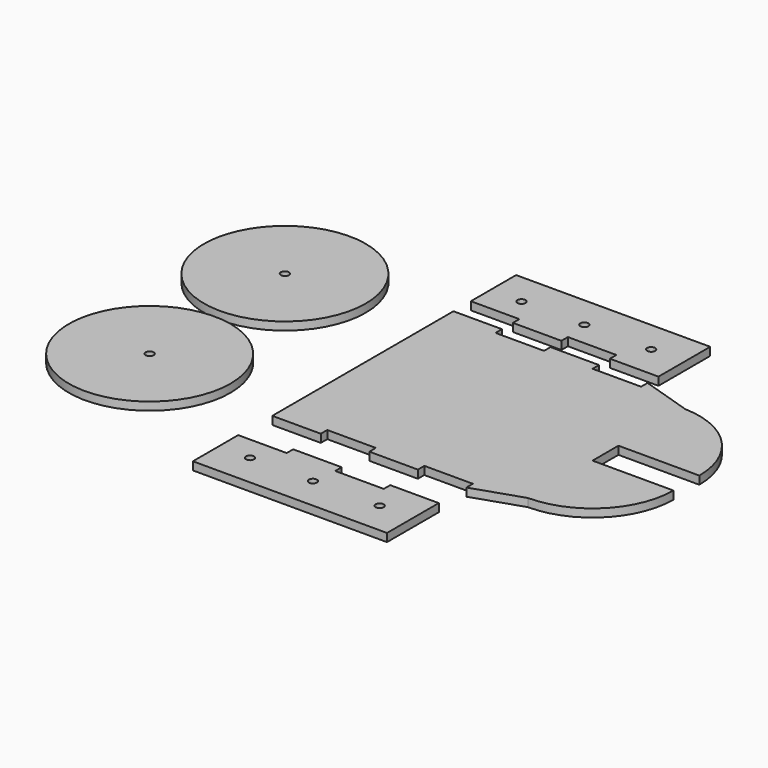
from build123d import *

# Parameters (mm, degrees)
F0_R     = 1.5875
F1_DEPTH = 3.175
F0_R_2   = 31.75


# Not quite as in the source:
# - a feature names something its author has since deleted; it is built from what else it names


with BuildPart() as f1:
    # F0 (on Top) → F1 (new body)
    with BuildSketch(Plane.XY):
        Polygon((19.05, 97.4367505789), (19.05, 94.2617505789), (38.1, 94.2617505789), (38.1, 97.4367505789), (57.15, 97.4367505789), (57.15, 94.2617505789), (76.2, 94.2617505789), (76.2, 119.6617505789), (50.8, 119.6617505789), (0, 119.6617505789), (0, 97.4367505789), align=None)
        with Locations((12.2715613582, 106.9617505789)):
            Circle(F0_R, mode=Mode.SUBTRACT)
        with Locations((36.9603613582, 106.9617505789)):
            Circle(F0_R, mode=Mode.SUBTRACT)
        with Locations((63.1541113582, 106.9617505789)):
            Circle(F0_R, mode=Mode.SUBTRACT)
    extrude(amount=F1_DEPTH)


with BuildPart() as f1b:
    # F0 (on Top) → F1, piece 2 (new body)
    with BuildSketch(Plane.XY):
        with BuildLine():
            Line((0, 88.9), (0, 0))
            Line((0, 0), (19.05, 0))
            Line((19.05, 0), (19.05, 3.175))
            Line((19.05, 3.175), (38.1, 3.175))
            Line((38.1, 3.175), (38.1, 0))
            Line((38.1, 0), (57.15, 0))
            Line((57.15, 0), (57.15, 3.175))
            Line((57.15, 3.175), (76.2, 3.175))
            Line((76.2, 3.175), (76.2, 0))
            Line((76.2, 0), (95.25, 6.35))
            ThreePointArc((95.25, 6.35), (117.7006403027, 15.6493596973), (127, 38.1))
            Line((127, 38.1), (95.25, 38.1))
            Line((95.25, 38.1), (95.25, 50.8))
            Line((95.25, 50.8), (127, 50.8))
            ThreePointArc((127, 50.8), (118.0154697598, 72.9313326895), (96.1467158039, 82.5373344937))
            Line((96.1467158039, 82.5373344937), (76.2, 88.9))
            Line((76.2, 88.9), (76.2, 85.725))
            Line((76.2, 85.725), (57.15, 85.725))
            Line((57.15, 85.725), (57.15, 88.9))
            Line((57.15, 88.9), (38.1, 88.9))
            Line((38.1, 88.9), (38.1, 85.725))
            Line((38.1, 85.725), (19.05, 85.725))
            Line((19.05, 85.725), (19.05, 88.9))
            Line((19.05, 88.9), (0, 88.9))
        make_face()
    extrude(amount=F1_DEPTH)


with BuildPart() as f1c:
    # F0 (on Top) → F1, piece 3 (new body)
    with BuildSketch(Plane.XY):
        with Locations((-55.9344552457, 76.1064253747)):
            Circle(F0_R_2)
        with Locations((-55.9344552457, 76.1064253747)):
            Circle(F0_R, mode=Mode.SUBTRACT)
    extrude(amount=F1_DEPTH)


with BuildPart() as f1d:
    # F0 (on Top) → F1, piece 4 (new body)
    with BuildSketch(Plane.XY):
        with Locations((-55.0876557827, 8.6811911315)):
            Circle(F0_R_2)
        with Locations((-55.0876557827, 8.6811911315)):
            Circle(F0_R, mode=Mode.SUBTRACT)
    extrude(amount=F1_DEPTH)


with BuildPart() as f1e:
    # F0 (on Top) → F1, piece 5 (new body)
    with BuildSketch(Plane.XY):
        Polygon((18.8933457804, -16.5366958239), (-0.1566542196, -16.5366958239), (-0.1566542196, -38.7616958239), (36.8386008513, -38.7616958239), (76.0433457804, -38.7616958239), (76.0433457804, -13.3616958239), (56.9933457804, -13.3616958239), (56.9933457804, -16.5366958239), (37.9433457804, -16.5366958239), (37.9433457804, -13.3616958239), (18.8933457804, -13.3616958239), align=None)
        with Locations((12.1149071386, -26.0616958239)):
            Circle(F0_R, mode=Mode.SUBTRACT)
        with Locations((36.8037071386, -26.0616958239)):
            Circle(F0_R, mode=Mode.SUBTRACT)
        with Locations((62.9974571386, -26.0616958239)):
            Circle(F0_R, mode=Mode.SUBTRACT)
    extrude(amount=F1_DEPTH)


solid = Compound([f1.part, f1b.part, f1c.part, f1d.part, f1e.part])
